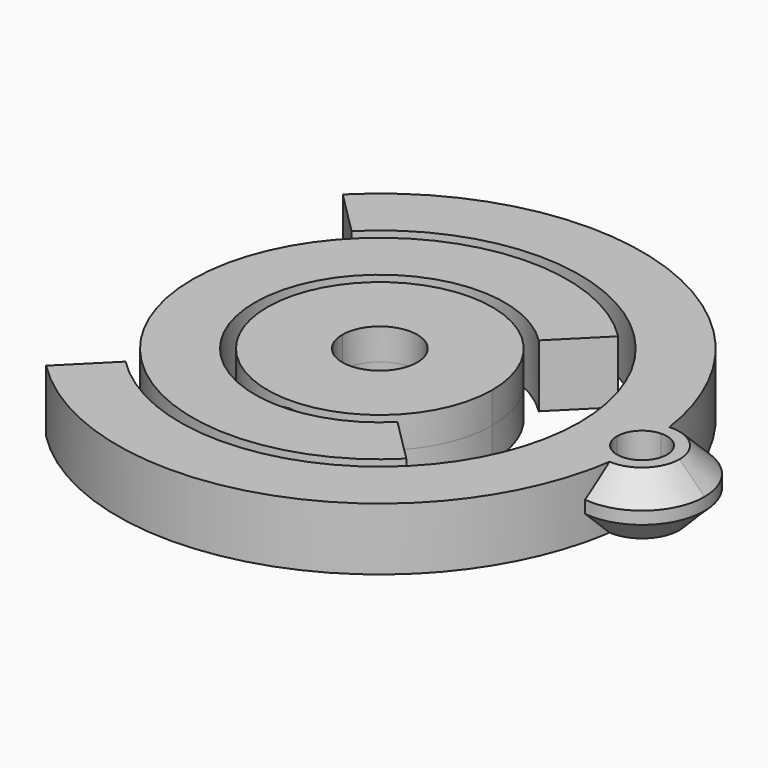
from build123d import *

# Parameters (mm, degrees)
F1_DEPTH = 2.5
F3_ANGLE = 135
F10_SIZE = 2


with BuildPart() as f1:
    # F0 (on Top) → F1 (new body, symmetric)
    with BuildSketch(Plane.XY):
        with BuildLine():
            ThreePointArc((-15, 0), (-5.7402514855, -13.8581929877), (10.6066017178, -10.6066017178))
            Line((10.6066017178, -10.6066017178), (7.0710678119, -7.0710678119))
            ThreePointArc((7.0710678119, -7.0710678119), (-3.8268343237, -9.2387953251), (-10, 0))
            Line((-10, 0), (-15, 0))
        make_face()
        with BuildLine():
            Line((7.0710678119, -7.0710678119), (10.6066017178, -10.6066017178))
            ThreePointArc((10.6066017178, -10.6066017178), (13.8581929877, -5.7402514855), (15, 0))
            ThreePointArc((15, 0), (10.6066017178, 10.6066017178), (0, 15))
            Line((0, 15), (0, 10))
            ThreePointArc((0, 10), (7.0710678119, 7.0710678119), (10, 0))
            ThreePointArc((10, 0), (9.2387953251, -3.8268343237), (7.0710678119, -7.0710678119))
        make_face()
    extrude(amount=F1_DEPTH, both=True)


with BuildPart() as f1b:
    # F0 (on Top) → F1, piece 2 (new body, symmetric)
    with BuildSketch(Plane.XY):
        with BuildLine():
            ThreePointArc((-6.3639610307, 6.3639610307), (-6.3639610307, -6.3639610307), (6.3639610307, -6.3639610307))
            Line((6.3639610307, -6.3639610307), (2.1213203436, -2.1213203436))
            ThreePointArc((2.1213203436, -2.1213203436), (-2.1213203436, -2.1213203436), (-2.1213203436, 2.1213203436))
            Line((-2.1213203436, 2.1213203436), (-6.3639610307, 6.3639610307))
        make_face()
        with BuildLine():
            Line((2.1213203436, -2.1213203436), (6.3639610307, -6.3639610307))
            ThreePointArc((6.3639610307, -6.3639610307), (8.3149157926, -3.4441508913), (9, 0))
            ThreePointArc((9, 0), (3.4441508913, 8.3149157926), (-6.3639610307, 6.3639610307))
            Line((-6.3639610307, 6.3639610307), (-2.1213203436, 2.1213203436))
            ThreePointArc((-2.1213203436, 2.1213203436), (1.1480502971, 2.7716385975), (3, 0))
            ThreePointArc((3, 0), (2.7716385975, -1.1480502971), (2.1213203436, -2.1213203436))
        make_face()
    extrude(amount=F1_DEPTH, both=True)


with BuildPart() as f1c:
    # F0 (on Top) → F1, piece 3 (new body, symmetric)
    with BuildSketch(Plane.XY):
        with BuildLine():
            ThreePointArc((-21, -4.6e-09), (-14.8492424033, -14.8492424065), (0, -21))
            Line((0, -21), (0, -16))
            ThreePointArc((0, -16), (-14.7820725201, -6.122934918), (-11.3137084992, 11.3137084988))
            ThreePointArc((-11.3137084992, 11.3137084988), (-14.5510928161, 9.8581396387), (-17.9387366299, 10.9179543928))
            ThreePointArc((-17.9387366299, 10.9179543928), (-20.2202060978, 5.6695030965), (-21, -4.6e-09))
        make_face()
        with BuildLine():
            Line((16, 0), (21, 0))
            ThreePointArc((21, 0), (14.8492424134, 14.8492423965), (2.39e-08, 21))
            ThreePointArc((2.39e-08, 21), (-5.6695030872, 20.2202061004), (-10.9179543928, 17.9387366299))
            ThreePointArc((-10.9179543928, 17.9387366299), (-10.1239678065, 16.4838004399), (-9.8492424049, 14.8492424049))
            ThreePointArc((-9.8492424049, 14.8492424049), (-10.2298447424, 12.935825243), (-11.3137084992, 11.3137084988))
            ThreePointArc((-11.3137084992, 11.3137084988), (6.1229349177, 14.7820725202), (16, 0))
        make_face()
        with BuildLine():
            ThreePointArc((-9.8492424049, 14.8492424049), (-10.1239678065, 16.4838004399), (-10.9179543928, 17.9387366299))
            ThreePointArc((-10.9179543928, 17.9387366299), (-12.1748979156, 17.1105774521), (-13.3692896663, 16.1945081376))
            ThreePointArc((-13.3692896663, 16.1945081376), (-12.9837792617, 15.5703854291), (-12.8492424049, 14.8492424049))
            ThreePointArc((-12.8492424049, 14.8492424049), (-13.0014833399, 14.0838755402), (-13.4350288425, 13.4350288425))
            Line((-13.4350288425, 13.4350288425), (-11.313708499, 11.313708499))
            ThreePointArc((-11.3137084992, 11.3137084988), (-10.2298447424, 12.935825243), (-9.8492424049, 14.8492424049))
        make_face()
        with BuildLine():
            ThreePointArc((-17.9387366299, 10.9179543928), (-14.5510928161, 9.8581396387), (-11.3137084992, 11.3137084988))
            Line((-11.313708499, 11.313708499), (-13.4350288425, 13.4350288425))
            ThreePointArc((-13.4350288425, 13.4350288425), (-14.8016098464, 12.8498097005), (-16.1945081376, 13.3692896663))
            ThreePointArc((-16.1945081376, 13.3692896663), (-17.1105774521, 12.1748979156), (-17.9387366299, 10.9179543928))
        make_face()
        with BuildLine():
            Line((-16.2634559673, 16.2634559673), (-18.3847763109, 18.3847763109))
            ThreePointArc((-18.3847763109, 18.3847763109), (-19.8403451711, 14.551092816), (-17.9387366299, 10.9179543928))
            ThreePointArc((-17.9387366299, 10.9179543928), (-17.1105774521, 12.1748979156), (-16.1945081376, 13.3692896663))
            ThreePointArc((-16.1945081376, 13.3692896663), (-16.8486751093, 14.8016098464), (-16.2634559673, 16.2634559673))
        make_face()
        with BuildLine():
            ThreePointArc((-13.3692896663, 16.1945081376), (-12.1748979156, 17.1105774521), (-10.9179543928, 17.9387366299))
            ThreePointArc((-10.9179543928, 17.9387366299), (-14.551092816, 19.8403451711), (-18.3847763109, 18.3847763109))
            Line((-18.3847763109, 18.3847763109), (-16.2634559673, 16.2634559673))
            ThreePointArc((-16.2634559673, 16.2634559673), (-14.8016098464, 16.8486751093), (-13.3692896663, 16.1945081376))
        make_face()
    extrude(amount=F1_DEPTH, both=True)


with BuildPart() as f1c_1:
    # F3: moved
    add(f1c.part.rotate(Axis((0, 0, 2.0642224699), (0, 0, -1)), F3_ANGLE))


with BuildPart() as f1_1:
    # F3: moved
    add(f1.part.rotate(Axis((0, 0, 2.0642224699), (0, 0, -1)), F3_ANGLE))

    # F4 (on Top) → F5, piece 2 (revolve)
    with BuildSketch(Plane.XY):
        Polygon((0, 17.7789945155), (0, 15.0089114904), (1.9535381021, 14.620516467), align=None)
        Polygon((0, -17.7789945155), (1.9535381021, -14.620516467), (0, -15.0089114904), align=None)
    revolve(axis=Axis((0, 16.393953003, 0), (0, 1, 0)))


with BuildPart() as f1b_1:
    # F3: moved
    add(f1b.part.rotate(Axis((0, 0, 2.0642224699), (0, 0, -1)), F3_ANGLE))

    # F4 (on Top) → F5 (revolve)
    with BuildSketch(Plane.XY):
        Polygon((0, 12.1097750962), (0, 9.0471189469), (2.2216387467, 8.5178322486), align=None)
        Polygon((0, -9.0471189469), (0, -12.1097750962), (2.2216387467, -8.5178322486), align=None)
    revolve(axis=Axis((0, 16.393953003, 0), (0, 1, 0)))


with BuildPart() as f7:
    # F6 (on Top) → F7 (revolve)
    with BuildSketch(Plane.XY):
        Polygon((0, 12.5458237512), (0, 9.0715390305), (2.3175082169, 8.5853263736), align=None)
    revolve(axis=Axis((0, 10.8086813908, 0), (0, 1, 0)))


with BuildPart() as f7b:
    # F6 (on Top) → F7, piece 2 (revolve)
    with BuildSketch(Plane.XY):
        Polygon((0, 18.2254966348), (0, 15.033331574), (2.0244383409, 14.7658399735), align=None)
    revolve(axis=Axis((0, 10.8086813908, 0), (0, 1, 0)))


with BuildPart() as f7c:
    # F6 (on Top) → F7, piece 3 (revolve)
    with BuildSketch(Plane.XY):
        Polygon((0, -9.0715390305), (0, -12.5458237512), (2.3175082169, -8.5853263736), align=None)
    revolve(axis=Axis((0, 10.8086813908, 0), (0, 1, 0)))


with BuildPart() as f7d:
    # F6 (on Top) → F7, piece 4 (revolve)
    with BuildSketch(Plane.XY):
        Polygon((2.0244383409, -14.7658399735), (0, -15.033331574), (0, -18.2254966348), align=None)
    revolve(axis=Axis((0, 10.8086813908, 0), (0, 1, 0)))


with BuildPart() as f1c_2:
    add(f1c_1.part)

    # F8: cut F7b, F7d
    add(f7b.part, mode=Mode.SUBTRACT)
    add(f7d.part, mode=Mode.SUBTRACT)

    # F10
    f10_edges = [f1c_2.edges().sort_by_distance(p)[0] for p in [
        (26, 0, 2.5),
        (26, 0, -2.5),
    ]]
    chamfer(f10_edges, length=F10_SIZE)


with BuildPart() as f1_2:
    add(f1_1.part)

    # F9: cut F7, F7c
    add(f7.part, mode=Mode.SUBTRACT)
    add(f7c.part, mode=Mode.SUBTRACT)


solid = Compound([f1b_1.part, f1c_2.part, f1_2.part])
